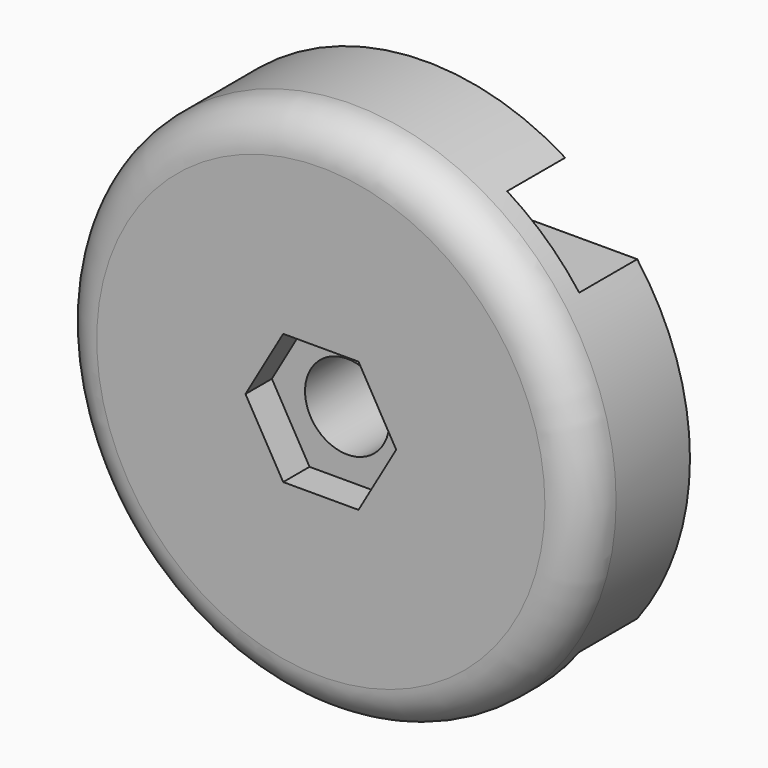
from build123d import *

# Parameters (mm, degrees)
F0_R          = 40
F1_DEPTH      = 20
F2_W          = 11
F2_H          = 10
F3_DEPTH      = 50
F3_DEPTH_BACK = 10
F4_R          = 6
F6_DEPTH      = 5
F7_R          = 6.4
F8_DEPTH      = 25


# Not quite as in the source:
# - a pattern or mirror of a feature is missing from the dataset's text; its kind, count and spacing are read off the source's solid


with BuildPart() as f1:
    # F0 (on Front) → F1 (new body)
    with BuildSketch(Plane.XZ):
        Circle(F0_R)
    extrude(amount=F1_DEPTH)

    # F2 (on Right) → F3 (cut, two sides)
    with BuildSketch(Plane.YZ) as f3_sk:
        with Locations((-5.5, 29)):
            Rectangle(F2_W, F2_H)
    f3 = extrude(amount=F3_DEPTH, mode=Mode.SUBTRACT) + extrude(f3_sk.sketch, amount=-F3_DEPTH_BACK, mode=Mode.SUBTRACT)

    # F3_copies: F3 across plane
    add(f3.mirror(Plane(origin=(0, 0, 0), x_dir=(-1, 0, 0), z_dir=(0, 0, -1))), mode=Mode.SUBTRACT)

    # F4
    f4_edges = [f1.edges().sort_by_distance(p)[0] for p in [
        (-40, -20, 0),
    ]]
    fillet(f4_edges, radius=F4_R)

    # F5 (on face) → F6 (cut)
    with BuildSketch(Plane.XZ.offset(20)):
        Polygon((-5.715767665, -9.9), (5.715767665, -9.9), (11.43153533, 0), (5.715767665, 9.9), (-5.715767665, 9.9), (-11.43153533, 0), align=None)
    extrude(amount=-F6_DEPTH, mode=Mode.SUBTRACT)

    # F7 (on face) → F8 (cut)
    with BuildSketch(Plane.XZ.offset(15)):
        Circle(F7_R)
    extrude(amount=-F8_DEPTH, mode=Mode.SUBTRACT)


solid = f1.part
